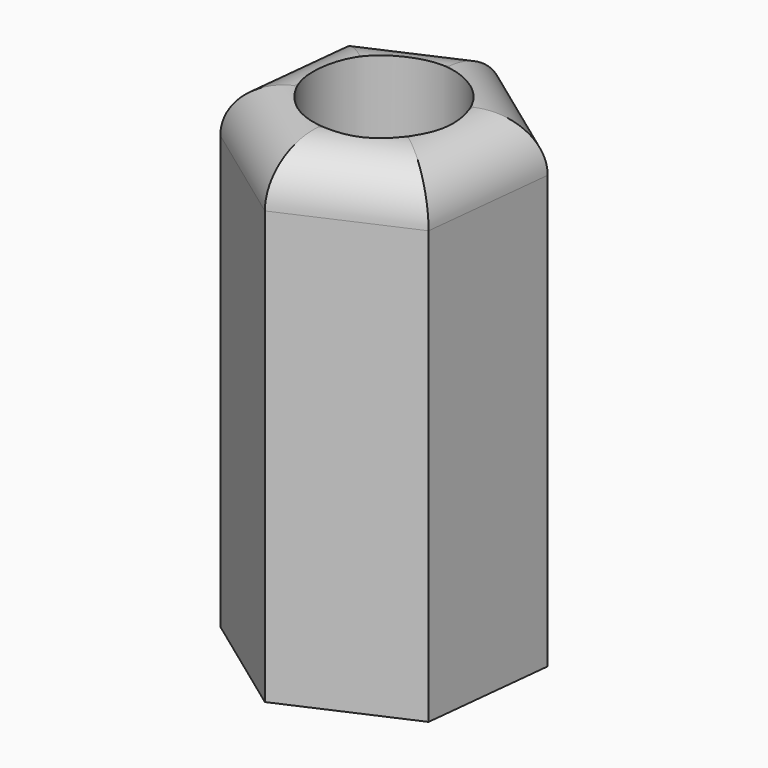
from build123d import *

# Parameters (mm, degrees)
F0_R         = 4.05
F1_DEPTH     = 28
F2_T1_DEPTH  = 22.6428048889
F2_T3_DEPTH  = 22.6428048889
F2_T5_DEPTH  = 22.6428048889
F2_T7_DEPTH  = 22.6428048889
F2_T9_DEPTH  = 22.6428048889
F2_T11_DEPTH = 22.6428048889


# Not quite as in the source:
# - a fillet or chamfer that OpenCascade refuses, or shapes differently, is made with other operations: its cross-section is extruded or revolved along the edge and cut away or added


with BuildPart() as f1:
    # F0 (on Top) → F1 (new body)
    with BuildSketch(Plane.XY):
        Polygon((6.1779160549, -4.4995355079), (6.9856700826, 3.1004644921), (0.8077540276, 7.6), (-6.1779160549, 4.4995355079), (-6.9856700826, -3.1004644921), (-0.8077540276, -7.6), align=None)
        Circle(F0_R, mode=Mode.SUBTRACT)
    extrude(amount=F1_DEPTH)

    # F2: fillet of radius 3 on 6 edges, made by hand

    # F2_s2 → F2_t1 (cut)
    with BuildSketch(Plane(origin=(-10.3479787197, -4.5927649325, 0), x_dir=(0, 0, 1), z_dir=(0.9140191571, 0.4056710249, 0))):
        with BuildLine():
            ThreePointArc((25, 6.6188631899), (27.1213203436, 5.7401835335), (28, 3.6188631899))
            Line((28, 3.6188631899), (28, 6.6188631899))
            Line((28, 6.6188631899), (25, 6.6188631899))
        make_face()
    extrude(amount=F2_T1_DEPTH, mode=Mode.SUBTRACT)

    # F2_s4 → F2_t3 (cut)
    with BuildSketch(Plane(origin=(-9.151440465, 6.6652299829, 0), x_dir=(0, 0, 1), z_dir=(0.8083309917, -0.5887282972, 0))):
        with BuildLine():
            ThreePointArc((25, 6.6188631899), (27.1213203436, 5.7401835335), (28, 3.6188631899))
            Line((28, 3.6188631899), (28, 6.6188631899))
            Line((28, 6.6188631899), (25, 6.6188631899))
        make_face()
    extrude(amount=F2_T3_DEPTH, mode=Mode.SUBTRACT)

    # F2_s6 → F2_t5 (cut)
    with BuildSketch(Plane(origin=(1.1965382547, 11.2579949153, 0), x_dir=(0, 0, 1), z_dir=(-0.1056881655, -0.994399322, 0))):
        with BuildLine():
            ThreePointArc((25, 6.6188631899), (27.1213203436, 5.7401835335), (28, 3.6188631899))
            Line((28, 3.6188631899), (28, 6.6188631899))
            Line((28, 6.6188631899), (25, 6.6188631899))
        make_face()
    extrude(amount=F2_T5_DEPTH, mode=Mode.SUBTRACT)

    # F2_s8 → F2_t7 (cut)
    with BuildSketch(Plane(origin=(10.3479787197, 4.5927649325, 0), x_dir=(0, 0, 1), z_dir=(-0.9140191571, -0.4056710249, 0))):
        with BuildLine():
            ThreePointArc((25, 6.6188631899), (27.1213203436, 5.7401835335), (28, 3.6188631899))
            Line((28, 3.6188631899), (28, 6.6188631899))
            Line((28, 6.6188631899), (25, 6.6188631899))
        make_face()
    extrude(amount=F2_T7_DEPTH, mode=Mode.SUBTRACT)

    # F2_s10 → F2_t9 (cut)
    with BuildSketch(Plane(origin=(9.151440465, -6.6652299829, 0), x_dir=(0, 0, 1), z_dir=(-0.8083309917, 0.5887282972, 0))):
        with BuildLine():
            ThreePointArc((25, 6.6188631899), (27.1213203436, 5.7401835335), (28, 3.6188631899))
            Line((28, 3.6188631899), (28, 6.6188631899))
            Line((28, 6.6188631899), (25, 6.6188631899))
        make_face()
    extrude(amount=F2_T9_DEPTH, mode=Mode.SUBTRACT)

    # F2_s12 → F2_t11 (cut)
    with BuildSketch(Plane(origin=(-1.1965382547, -11.2579949153, 0), x_dir=(0, 0, 1), z_dir=(0.1056881655, 0.994399322, 0))):
        with BuildLine():
            ThreePointArc((25, 6.6188631899), (27.1213203436, 5.7401835335), (28, 3.6188631899))
            Line((28, 3.6188631899), (28, 6.6188631899))
            Line((28, 6.6188631899), (25, 6.6188631899))
        make_face()
    extrude(amount=F2_T11_DEPTH, mode=Mode.SUBTRACT)


solid = f1.part
